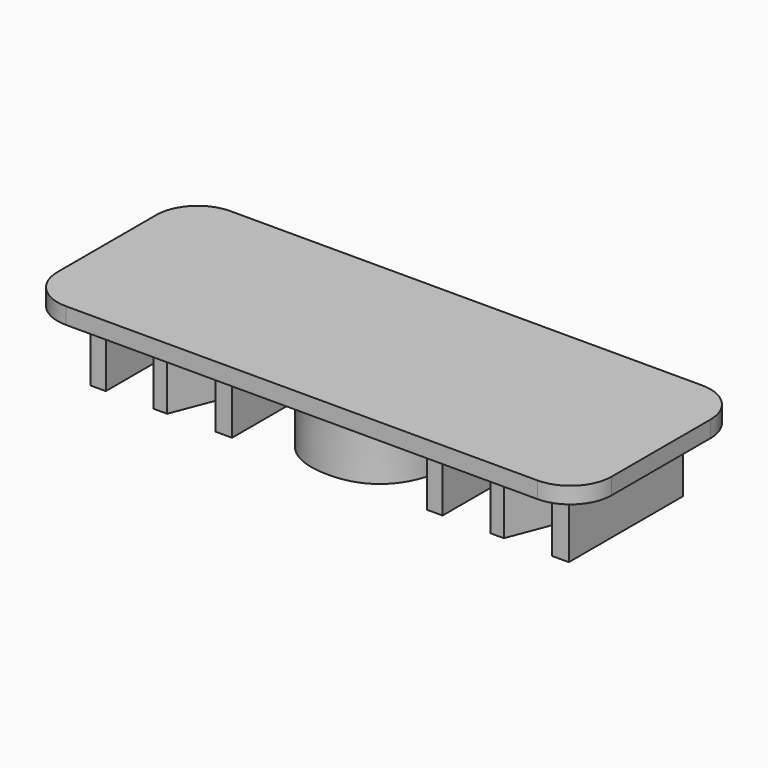
from build123d import *

# Parameters (mm, degrees)
F0_TEXT_SIZE = 30.8912396275
F1_DEPTH     = 10.16
F2_W         = 85.4585228352
F2_H         = 31.75
F3_DEPTH     = 2.54
F4_R         = 6.35


# Not quite as in the source:
# - Text() gives the source's letters only with a copy of the font that has no kerning and outlines rounded to 1/6400 em; it was checked with that copy


with BuildPart() as f1:
    # F0 (on Top) → F1 (new body)
    with BuildSketch(Plane.XY):
        with Locations((-39.4104643061, -11.1252)):
            Text('MOM', F0_TEXT_SIZE, font='Open Sans', text_align=(TextAlign.LEFT, TextAlign.BOTTOM))
    extrude(amount=-F1_DEPTH)


with BuildPart() as f3:
    # F2 (on Top) → F3 (new body)
    with BuildSketch(Plane.XY):
        Rectangle(F2_W, F2_H)
    extrude(amount=F3_DEPTH)

    # F4
    f4_edges = [f3.edges().sort_by_distance(p)[0] for p in [
        (-42.729261, -15.875, 1.27),
        (-42.729261, 15.875, 1.27),
        (42.729261, 15.875, 1.27),
        (42.729261, -15.875, 1.27),
    ]]
    fillet(f4_edges, radius=F4_R)


solid = Compound([f1.part, f3.part])
